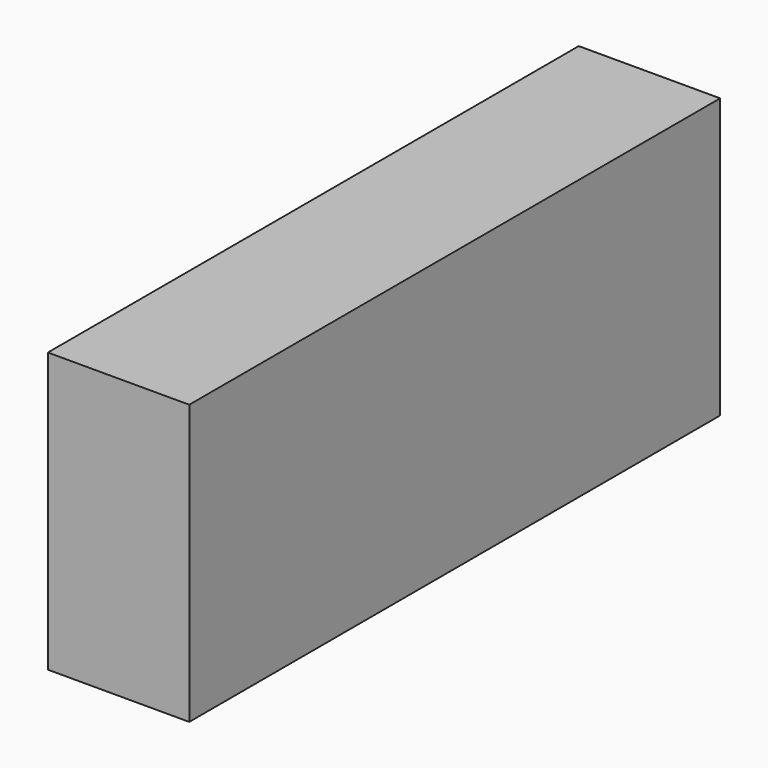
from build123d import *

# Parameters (mm, degrees)
F0_W      = 728.5054326057
F0_H      = 306.5502718091
F1_DEPTH  = 155.222194
F2_R      = 50.8
F3_DEPTH  = 7.62
F1_FACE_W = 728.5054326057
F1_FACE_H = 306.5502718091
F4_DEPTH  = 1191


# Not quite as in the source:
# - an extrude ends at something that could not be found from the text; its depth is read off the source's solid
# - a feature names something its author has since deleted; it is built from what else it names


with BuildPart() as f1:
    # F0 (on Right) → F1 (new body)
    with BuildSketch(Plane.YZ):
        with Locations((364.2527163029, -99.0724824369)):
            Rectangle(F0_W, F0_H)
    extrude(amount=F1_DEPTH)

    # F2 (on face) → F3 (join)
    with BuildSketch(Plane(origin=(0, 0, 0), x_dir=(0, -1, 0), z_dir=(-1, 0, 0))):
        with Locations((-335.2750743124, -123.5973465323)):
            Circle(F2_R)
    extrude(amount=-F3_DEPTH)

    # F2 (on face) + F1_face (on face) → F4 (cut, through all)
    with BuildSketch(Plane(origin=(0, 0, 0), x_dir=(0, -1, 0), z_dir=(-1, 0, 0))):
        with Locations((-335.2750743124, -123.5973465323)):
            Circle(F2_R)
    with BuildSketch(Plane(origin=(0, 364.2527163029, -99.0724824369), x_dir=(0, 1, 0), z_dir=(-1, 0, 0))):
        Rectangle(F1_FACE_W, F1_FACE_H)
    extrude(amount=F4_DEPTH, mode=Mode.SUBTRACT)


solid = f1.part
